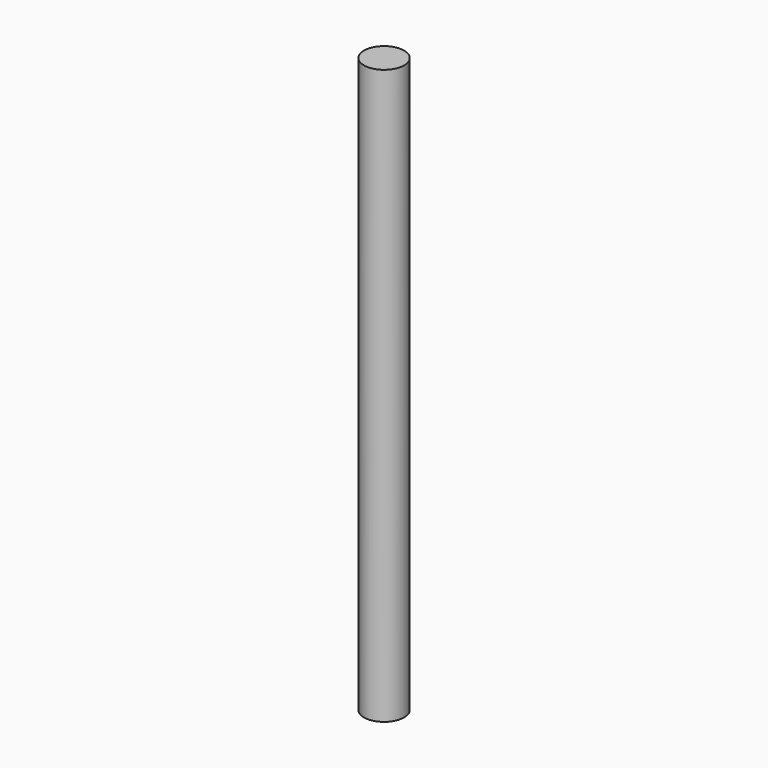
from build123d import *

# Parameters (mm, degrees)
F0_R     = 5.25
F1_DEPTH = 150


# Not quite as in the source:
# - a feature of the source that left no trace in its solid (it failed there, or was rolled back) is left out


with BuildPart() as f1:
    # F0 (on Top) → F1 (new body)
    with BuildSketch(Plane.XY):
        Circle(F0_R)
    extrude(amount=F1_DEPTH)


solid = f1.part
